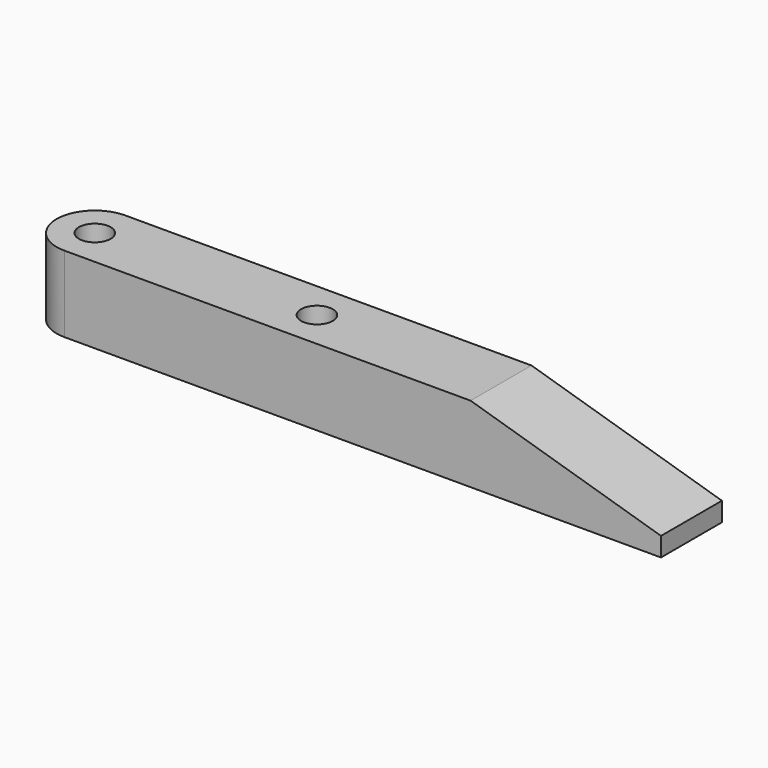
from build123d import *

# Parameters (mm, degrees)
F0_W     = 100
F0_H     = 12
F1_DEPTH = 12
F2_SIZE2 = 9
F2_SIZE  = 30
F3_R     = 5.99999
F5_D     = 5


# Not quite as in the source:
# - a fillet or chamfer is up to 0.001 mm smaller than in the source, because OpenCascade refuses the exact size


with BuildPart() as f1:
    # F0 (on Top) → F1 (new body)
    with BuildSketch(Plane.XY):
        with Locations((50, 6)):
            Rectangle(F0_W, F0_H)
    extrude(amount=F1_DEPTH)

    # F2
    f2_edges = [f1.edges().sort_by_distance(p)[0] for p in [
        (100, 6, 12),
    ]]
    f2_side = f1.faces().sort_by_distance((50, 6, 12))[0]
    chamfer(f2_edges, length=F2_SIZE, length2=F2_SIZE2, reference=f2_side)

    # F3 (radius 6 in the source; OpenCascade refuses exactly that, so slightly less here)
    f3_edges = [f1.edges().sort_by_distance(p)[0] for p in [
        (0, 0, 6),
        (0, 12, 6),
    ]]
    fillet(f3_edges, radius=F3_R)

    # F5 (through all)
    with Locations(Plane.XY.offset(12)):
        with Locations((6, 6), (41, 6)):
            Hole(F5_D / 2)


solid = f1.part
